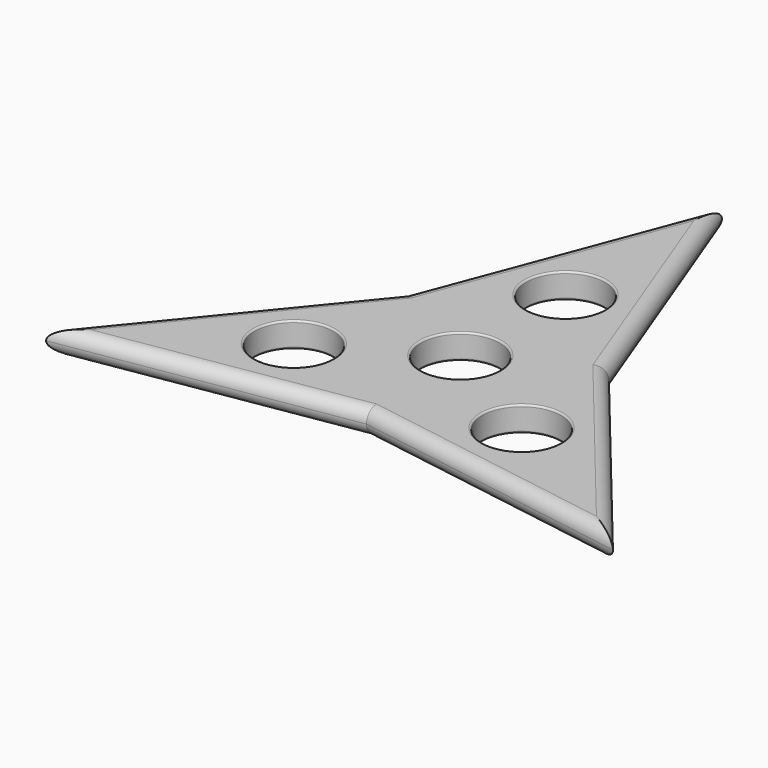
from build123d import *

# Parameters (mm, degrees)
F0_R     = 11
F1_DEPTH = 7
F2_R     = 3.5
F3_R     = 3.49999
F4_R     = 0.5
F5_R     = 0.5


# Not quite as in the source:
# - a fillet or chamfer is up to 0.001 mm smaller than in the source, because OpenCascade refuses the exact size


with BuildPart() as f1:
    # F0 (on Top) → F1 (new body)
    with BuildSketch(Plane.XY):
        Polygon((0.0125008091, -32.7994597757), (79.1922360659, -45.681424439), (28.3989149916, 16.4105559061), (-0.0348439877, 91.423200435), (-28.4114158007, 16.3889038696), (-79.1573920781, -45.7417759961), align=None)
        with Locations((-31.8169734902, -18.3695382094)):
            Circle(F0_R, mode=Mode.SUBTRACT)
        Circle(F0_R, mode=Mode.SUBTRACT)
        with Locations((31.8169734902, -18.3695382094)):
            Circle(F0_R, mode=Mode.SUBTRACT)
        with Locations((0, 36.7390764187)):
            Circle(F0_R, mode=Mode.SUBTRACT)
    extrude(amount=F1_DEPTH)

    # F2
    f2_edges = [f1.edges().sort_by_distance(p)[0] for p in [
        (-53.784404, -14.676436, 7),
        (-39.572446, -39.270618, 7),
        (-14.22313, 53.906052, 7),
        (14.182036, 53.916878, 7),
        (53.795576, -14.635434, 7),
        (39.602368, -39.240442, 7),
    ]]
    fillet(f2_edges, radius=F2_R)

    # F3 (radius 3.5 in the source; OpenCascade refuses exactly that, so slightly less here)
    f3_edges = [f1.edges().sort_by_distance(p)[0] for p in [
        (-14.22313, 53.906052, 0),
        (-53.784404, -14.676436, 0),
        (-39.572446, -39.270618, 0),
        (39.602368, -39.240442, 0),
        (53.795576, -14.635434, 0),
        (14.182036, 53.916878, 0),
    ]]
    fillet(f3_edges, radius=F3_R)

    # F4
    f4_edges = [f1.edges().sort_by_distance(p)[0] for p in [
        (20.816973, -18.369538, 7),
        (-11, 0, 7),
        (-42.816973, -18.369538, 7),
        (-11, 36.739076, 7),
    ]]
    fillet(f4_edges, radius=F4_R)

    # F5
    f5_edges = [f1.edges().sort_by_distance(p)[0] for p in [
        (20.816973, -18.369538, 0),
        (-11, 0, 0),
        (-11, 36.739076, 0),
        (-42.816973, -18.369538, 0),
    ]]
    fillet(f5_edges, radius=F5_R)


solid = f1.part
